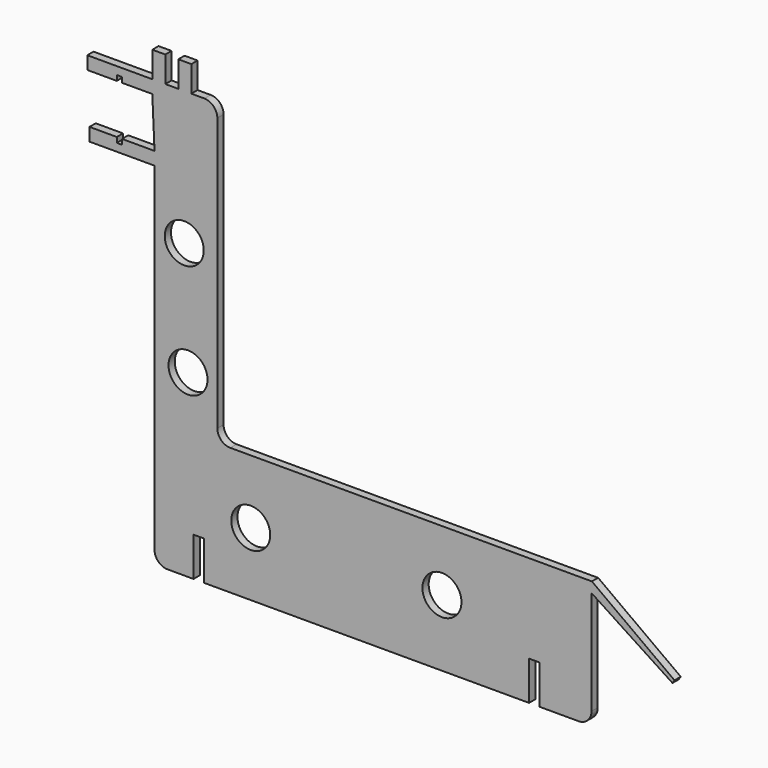
from build123d import *

# Parameters (mm, degrees)
F0_R     = 7.5
F1_DEPTH = 3
F2_R     = 5
F3_R     = 5
F4_R     = 5
F5_R     = 5


# Not quite as in the source:
# - a feature of the source that left no trace in its solid (it failed there, or was rolled back) is left out


with BuildPart() as f1:
    # F0 (on Front) → F1 (new body)
    with BuildSketch(Plane.XZ):
        Polygon((-45.7000464201, 51.51183635), (-70.7000464201, 51.51183635), (-70.7000464201, 46.51183635), (-63.6224076152, 46.51183635), (-59.3452238418, 46.51183635), (-59.3452238418, 48.51183635), (-57.3452238418, 48.51183635), (-57.3452238418, 46.51183635), (-45.7000464201, 46.51183635), (-44.8452238418, 27.5310756076), (-57.3452238418, 27.5310756076), (-57.3452238418, 25.5310756076), (-59.3452238418, 25.5310756076), (-59.3452238418, 27.5310756076), (-69.8452238418, 27.5310756076), (-69.8452238418, 22.5310756076), (-44.8452238418, 22.5310756076), (-44.8452238418, -112.4689243924), (-29.8452238418, -112.4689243924), (-29.8452238418, -97.4689243924), (-25.8452238418, -97.4689243924), (-25.8452238418, -112.4689243924), (99.1547761582, -112.4689243924), (99.1547761582, -97.4689243924), (103.1547761582, -97.4689243924), (103.1547761582, -112.4689243924), (123.1547761582, -112.4689243924), (123.1547761582, -67.4689243924), (154.2856724769, -87.808891194), (155.0577331575, -86.6272304158), (123.2999535799, -63.48816365), (-20.7000464201, -63.48816365), (-20.7000464201, 51.51183635), (-30.7000464201, 51.51183635), (-30.7000464201, 61.51183635), (-35.7000464201, 61.51183635), (-35.7000464201, 51.51183635), (-40.7000464201, 51.51183635), (-40.7000464201, 61.51183635), (-45.7000464201, 61.51183635), align=None)
        with Locations((-7.8524835408, -88.0068540573)):
            Circle(F0_R, mode=Mode.SUBTRACT)
        with Locations((-31.9686569273, -43.2611815631)):
            Circle(F0_R, mode=Mode.SUBTRACT)
        with Locations((65.6582638621, -86.8446305394)):
            Circle(F0_R, mode=Mode.SUBTRACT)
        with Locations((-33.4214381874, 0)):
            Circle(F0_R, mode=Mode.SUBTRACT)
    extrude(amount=F1_DEPTH)

    # F2
    f2_edges = [f1.edges().sort_by_distance(p)[0] for p in [
        (-20.700046, -1.5, 51.511836),
    ]]
    fillet(f2_edges, radius=F2_R)

    # F3
    f3_edges = [f1.edges().sort_by_distance(p)[0] for p in [
        (123.154776, -1.5, -112.468924),
    ]]
    fillet(f3_edges, radius=F3_R)

    # F4
    f4_edges = [f1.edges().sort_by_distance(p)[0] for p in [
        (-44.845224, -1.5, -112.468924),
    ]]
    fillet(f4_edges, radius=F4_R)

    # F5
    f5_edges = [f1.edges().sort_by_distance(p)[0] for p in [
        (-20.700046, -1.5, -63.488164),
    ]]
    fillet(f5_edges, radius=F5_R)


solid = f1.part
